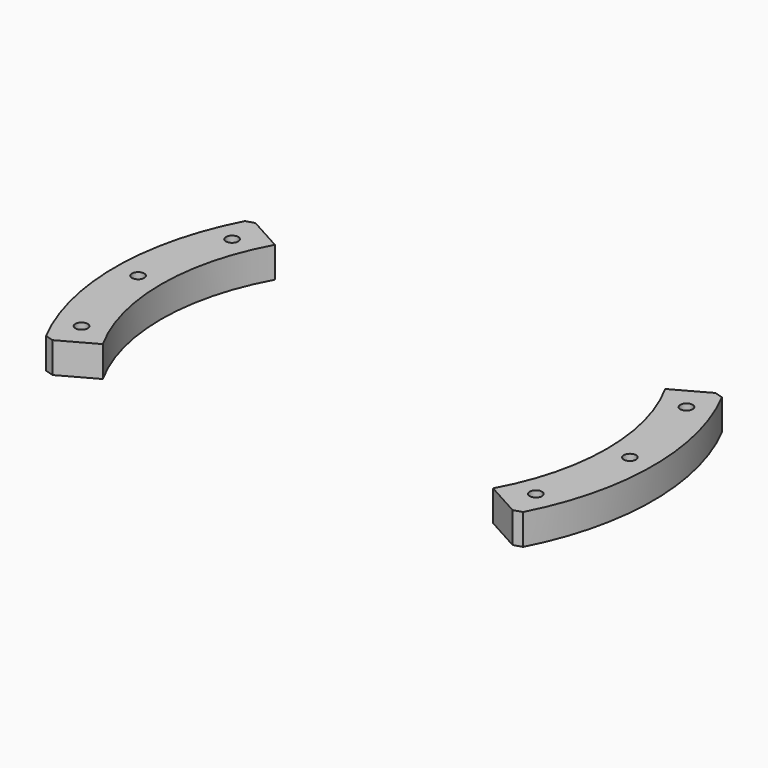
from build123d import *

# Parameters (mm, degrees)
F0_R        = 2
F1_DEPTH    = 10
F2_T1_DEPTH = 20.5212634911


# Not quite as in the source:
# - a fillet or chamfer that OpenCascade refuses, or shapes differently, is made with other operations: its cross-section is extruded or revolved along the edge and cut away or added


with BuildPart() as f1:
    # F0 (on Top) → F1 (new body)
    with BuildSketch(Plane.XY):
        with BuildLine():
            ThreePointArc((-63.492125496, -35), (-72.5, 0), (-63.492125496, 35))
            Line((-63.492125496, 35), (-76.6284273228, 42.2413793103))
            ThreePointArc((-76.6284273228, 42.2413793103), (-87.5, 0), (-76.6284273228, -42.2413793103))
            Line((-76.6284273228, -42.2413793103), (-63.492125496, -35))
        make_face()
        with Locations((-73.9103626009, -30.6146745892)):
            Circle(F0_R, mode=Mode.SUBTRACT)
        with Locations((-80, 0)):
            Circle(F0_R, mode=Mode.SUBTRACT)
        with Locations((-73.9103626009, 30.6146745892)):
            Circle(F0_R, mode=Mode.SUBTRACT)
    extrude(amount=F1_DEPTH)

    # F2: chamfer of 2 on 2 edges, made by hand

    # F2_s2 → F2_t1 (cut)
    with BuildSketch(Plane.XY.offset(-5.2606317456)):
        with BuildLine():
            Line((-74.8564321485, 41.2645679245), (-77.5955622411, 40.4373431432))
            ThreePointArc((-77.5955622411, 40.4373431432), (-77.1306266641, 41.3172655242), (-76.6284273228, 42.2413793103))
            Line((-76.6284273228, 42.2413793103), (-74.8564321485, 41.2645679245))
        make_face()
        with BuildLine():
            Line((-74.8564321485, -41.2645679245), (-77.5955622411, -40.4373431432))
            ThreePointArc((-77.5955622411, -40.4373431432), (-77.1306266641, -41.3172655242), (-76.6284273228, -42.2413793103))
            Line((-76.6284273228, -42.2413793103), (-74.8564321485, -41.2645679245))
        make_face()
    extrude(amount=F2_T1_DEPTH, mode=Mode.SUBTRACT)


with BuildPart() as f3_1:
    # F3: instance of F1
    add(f1.part.mirror(Plane.YZ))


solid = Compound([f1.part, f3_1.part])
